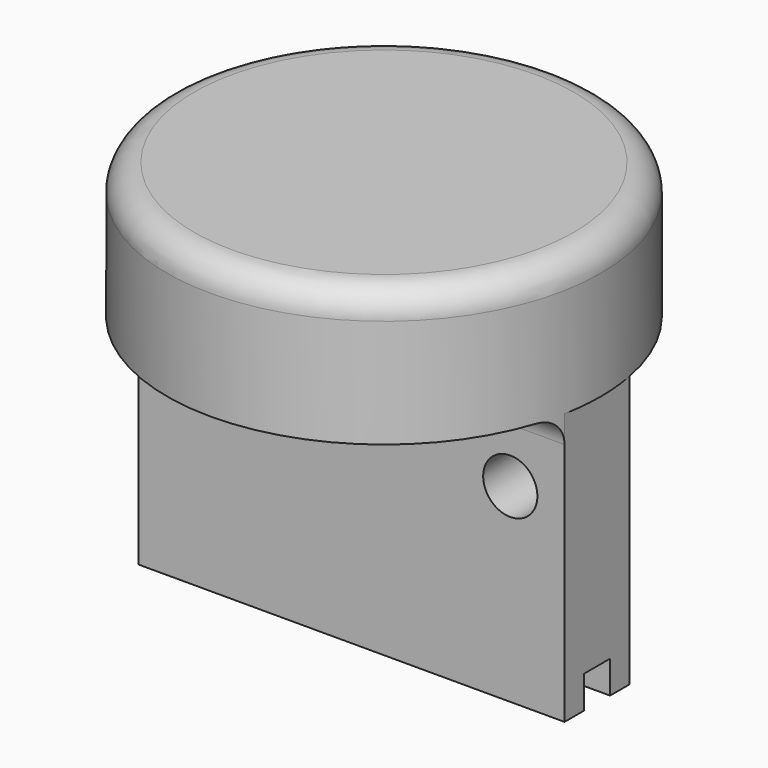
from build123d import *

# Parameters (mm, degrees)
F0_R        = 40
F1_DEPTH    = 25
F2_W        = 78.5811682275
F2_H        = 15
F3_DEPTH    = 50
F4_W        = 6
F4_H        = 12
F5_DEPTH    = 79.2915841138
F6_R        = 5
F7_DEPTH    = 25
F8_T4_DEPTH = 78.5811682275
F8_S5_R     = 40
F8_T6_DEPTH = 41


# Not quite as in the source:
# - a fillet or chamfer that OpenCascade refuses, or shapes differently, is made with other operations: its cross-section is extruded or revolved along the edge and cut away or added


with BuildPart() as f1:
    # F0 (on Top) → F1 (new body)
    with BuildSketch(Plane.XY):
        Circle(F0_R)
    extrude(amount=-F1_DEPTH)

    # F2 (on face) → F3 (join)
    with BuildSketch(Plane(origin=(0, 0, -25), x_dir=(1, 0, 0), z_dir=(0, 0, -1))):
        Rectangle(F2_W, F2_H)
    extrude(amount=F3_DEPTH)

    # F4 (on face) → F5 (cut, through all)
    with BuildSketch(Plane(origin=(-39.2905841138, 0, 0), x_dir=(0, -1, 0), z_dir=(-1, 0, 0))):
        with Locations((0, -75)):
            Rectangle(F4_W, F4_H)
    extrude(amount=-F5_DEPTH, mode=Mode.SUBTRACT)

    # F6 (on face) → F7 (cut)
    with BuildSketch(Plane(origin=(0, 7.5, 0), x_dir=(-1, 0, 0), z_dir=(0, 1, 0))):
        with Locations((-29.2905841138, -40)):
            Circle(F6_R)
        with Locations((29.2905841138, -40)):
            Circle(F6_R)
    extrude(amount=-F7_DEPTH, mode=Mode.SUBTRACT)

    # F8: fillet of radius 5 on 2 edges, made by hand


with BuildPart() as f8_tool2:
    # F8_s3 → F8_t4 (new body)
    with BuildSketch(Plane.YZ.offset(39.2905841138)):
        with BuildLine():
            ThreePointArc((-12.5, -25), (-8.9644660941, -26.4644660941), (-7.5, -30))
            Line((-7.5, -30), (-7.5, -25))
            Line((-7.5, -25), (-12.5, -25))
        make_face()
    extrude(amount=-F8_T4_DEPTH)

    # F8_s5 → F8_t6 (intersect, symmetric)
    with BuildSketch(Plane.XY.offset(-27.5)):
        Circle(F8_S5_R)
    extrude(amount=F8_T6_DEPTH, both=True, mode=Mode.INTERSECT)


with BuildPart() as f1_1:
    add(f1.part)

    # F8_t1: union F8_tool2
    add(f8_tool2.part)

    # F8_s7 → F8_t8 (revolve, cut)
    with BuildSketch(Plane.XZ):
        with BuildLine():
            ThreePointArc((40, -5), (38.5355339059, -1.4644660941), (35, 0))
            Line((35, 0), (40, 0))
            Line((40, 0), (40, -5))
        make_face()
    revolve(axis=Axis((0, 0, 0), (0, 0, 1)), mode=Mode.SUBTRACT)


solid = f1_1.part
